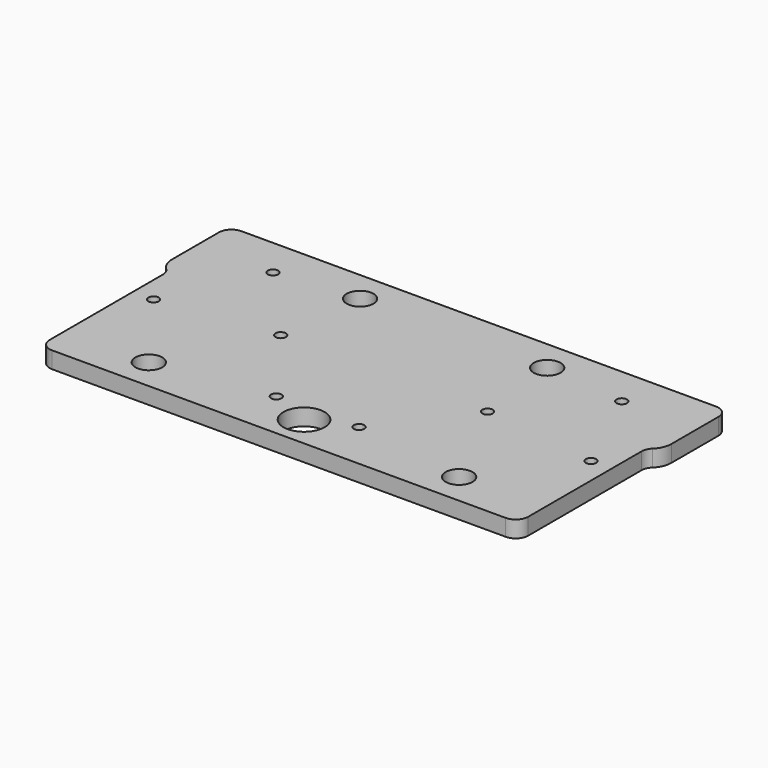
from build123d import *

# Parameters (mm, degrees)
F0_R         = 3.225
F0_R_2       = 1.25
F0_R_3       = 4.95
F1_DEPTH     = 4
F2_T1_DEPTH  = 4
F2_T3_DEPTH  = 4
F2_T5_DEPTH  = 19
F2_T7_DEPTH  = 19
F2_T9_DEPTH  = 19
F2_T11_DEPTH = 19
F3_R         = 5


# Not quite as in the source:
# - a fillet or chamfer that OpenCascade refuses, or shapes differently, is made with other operations: its cross-section is extruded or revolved along the edge and cut away or added


with BuildPart() as f1:
    # F0 (on Top) → F1 (new body)
    with BuildSketch(Plane.XY):
        Polygon((60, 10), (60, 30), (-60, 30), (-60, 10), (-57.5, 10), (-57.5, -30), (57.5, -30), (57.5, 10), align=None)
        with Locations((-37.275, -22.475)):
            Circle(F0_R, mode=Mode.SUBTRACT)
        with Locations((-9.95, -18.35)):
            Circle(F0_R_2, mode=Mode.SUBTRACT)
        with Locations((-52.55, -1.95)):
            Circle(F0_R_2, mode=Mode.SUBTRACT)
        with Locations((0, -22.45)):
            Circle(F0_R_3, mode=Mode.SUBTRACT)
        with Locations((9.95, -18.35)):
            Circle(F0_R_2, mode=Mode.SUBTRACT)
        with Locations((37.275, -22.475)):
            Circle(F0_R, mode=Mode.SUBTRACT)
        with Locations((52.55, -1.95)):
            Circle(F0_R_2, mode=Mode.SUBTRACT)
        with Locations((-24.85, 1.6)):
            Circle(F0_R_2, mode=Mode.SUBTRACT)
        with Locations((-41.9, 20.6)):
            Circle(F0_R_2, mode=Mode.SUBTRACT)
        with Locations((-22.475, 22.475)):
            Circle(F0_R, mode=Mode.SUBTRACT)
        with Locations((24.85, 1.6)):
            Circle(F0_R_2, mode=Mode.SUBTRACT)
        with Locations((22.475, 22.475)):
            Circle(F0_R, mode=Mode.SUBTRACT)
        with Locations((41.9, 20.6)):
            Circle(F0_R_2, mode=Mode.SUBTRACT)
    extrude(amount=F1_DEPTH)

    # F2: fillet of radius 3 on 6 edges, made by hand

    # F2_s2 → F2_t1 (join)
    with BuildSketch(Plane.XY):
        with BuildLine():
            ThreePointArc((-60, 10), (-58.2087121525, 8.9784517816), (-57.5, 7.0419601084))
            Line((-57.5, 7.0419601084), (-57.5, 10))
            Line((-57.5, 10), (-60, 10))
        make_face()
    extrude(amount=F2_T1_DEPTH)

    # F2_s4 → F2_t3 (join)
    with BuildSketch(Plane.XY):
        with BuildLine():
            ThreePointArc((60, 10), (58.2087121525, 8.9784517816), (57.5, 7.0419601084))
            Line((57.5, 7.0419601084), (57.5, 10))
            Line((57.5, 10), (60, 10))
        make_face()
    extrude(amount=F2_T3_DEPTH)

    # F2_s6 → F2_t5 (cut)
    with BuildSketch(Plane.XY.offset(-7.5)):
        with BuildLine():
            ThreePointArc((60, 27), (59.1213203436, 29.1213203436), (57, 30))
            Line((57, 30), (60, 30))
            Line((60, 30), (60, 27))
        make_face()
    extrude(amount=F2_T5_DEPTH, mode=Mode.SUBTRACT)

    # F2_s8 → F2_t7 (cut)
    with BuildSketch(Plane.XY.offset(-7.5)):
        with BuildLine():
            ThreePointArc((-60, 27), (-59.1213203436, 29.1213203436), (-57, 30))
            Line((-57, 30), (-60, 30))
            Line((-60, 30), (-60, 27))
        make_face()
    extrude(amount=F2_T7_DEPTH, mode=Mode.SUBTRACT)

    # F2_s10 → F2_t9 (cut)
    with BuildSketch(Plane.XY.offset(-7.5)):
        with BuildLine():
            ThreePointArc((-54.5, -30), (-56.6213203436, -29.1213203436), (-57.5, -27))
            Line((-57.5, -27), (-57.5, -30))
            Line((-57.5, -30), (-54.5, -30))
        make_face()
    extrude(amount=F2_T9_DEPTH, mode=Mode.SUBTRACT)

    # F2_s12 → F2_t11 (cut)
    with BuildSketch(Plane.XY.offset(-7.5)):
        with BuildLine():
            ThreePointArc((57.5, -27), (56.6213203436, -29.1213203436), (54.5, -30))
            Line((54.5, -30), (57.5, -30))
            Line((57.5, -30), (57.5, -27))
        make_face()
    extrude(amount=F2_T11_DEPTH, mode=Mode.SUBTRACT)

    # F3
    f3_edges = [f1.edges().sort_by_distance(p)[0] for p in [
        (-60, 10, 2),
        (60, 10, 2),
    ]]
    fillet(f3_edges, radius=F3_R)


solid = f1.part
